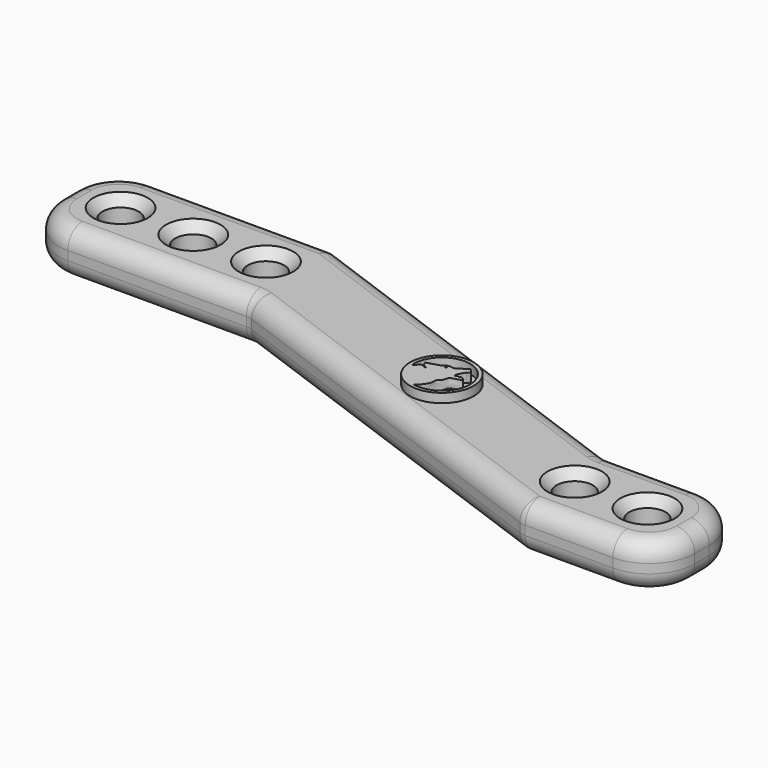
from build123d import *

# Parameters (mm, degrees)
F0_W         = 25
F0_H         = 12
F0_W_2       = 15
F1_DEPTH     = 5
F2_R         = 2
F3_DEPTH     = 5.001
F4_R         = 2
F5_T1_DEPTH  = 5
F5_T4_ANGLE  = 90
F5_T6_ANGLE  = 90
F5_T8_ANGLE  = 90
F5_T10_ANGLE = 90
F5_T12_ANGLE = 90
F5_T14_ANGLE = 90
F5_T16_ANGLE = 90
F5_T18_ANGLE = 90
F6_SIZE      = 1
F8_DEPTH     = 1


# Not quite as in the source:
# - a fillet or chamfer that OpenCascade refuses, or shapes differently, is made with other operations: its cross-section is extruded or revolved along the edge and cut away or added


with BuildPart() as f1:
    # F0 (on Top) → F1 (new body)
    with BuildSketch(Plane.XY):
        with Locations((12.5, 6)):
            Rectangle(F0_W, F0_H)
        with Locations((74.7861679354, -9.3909064497)):
            Rectangle(F0_W_2, F0_H)
        Polygon((25, 12), (25, 0), (67.2861679354, -15.3909064497), (67.2861679354, -3.3909064497), align=None)
    extrude(amount=F1_DEPTH)

    # F2 (on face) → F3 (cut, through all)
    with BuildSketch(Plane.XY.offset(5)):
        with Locations((6, 6)):
            Circle(F2_R)
        with Locations((14, 6)):
            Circle(F2_R)
        with Locations((22, 6)):
            Circle(F2_R)
        with Locations((68.2861679354, -9.3909064497)):
            Circle(F2_R)
        with Locations((76.2861679354, -9.3909064497)):
            Circle(F2_R)
    extrude(amount=-F3_DEPTH, mode=Mode.SUBTRACT)

    # F4
    f4_edges = [f1.edges().sort_by_distance(p)[0] for p in [
        (12.5, 12, 5),
        (12.5, 12, 0),
        (0, 6, 5),
        (0, 6, 0),
        (12.5, 0, 5),
        (12.5, 0, 0),
        (46.143084, -7.695453, 5),
        (74.786168, -15.390906, 5),
        (46.143084, -7.695453, 0),
        (74.786168, -15.390906, 0),
        (82.286168, -9.390906, 5),
        (82.286168, -9.390906, 0),
        (74.786168, -3.390906, 0),
        (74.786168, -3.390906, 5),
        (46.143084, 4.304547, 5),
        (46.143084, 4.304547, 0),
        (25, 12, 2.5),
        (67.286168, -3.390906, 2.5),
        (67.286168, -15.390906, 2.5),
        (25, 0, 2.5),
    ]]
    fillet(f4_edges, radius=F4_R)

    # F5: fillet of radius 5 on 6 edges, made by hand

    # F5_s2 → F5_t1 (cut)
    with BuildSketch(Plane.XY):
        with BuildLine():
            ThreePointArc((0, 5), (1.4644660941, 1.4644660941), (5, 0))
            Line((5, 0), (0, 0))
            Line((0, 0), (0, 5))
        make_face()
        with BuildLine():
            ThreePointArc((82.2861679354, -10.3909064497), (80.8217018413, -13.9264403556), (77.2861679354, -15.3909064497))
            Line((77.2861679354, -15.3909064497), (82.2861679354, -15.3909064497))
            Line((82.2861679354, -15.3909064497), (82.2861679354, -10.3909064497))
        make_face()
        with BuildLine():
            ThreePointArc((77.2861679354, -3.3909064497), (80.8217018413, -4.8553725437), (82.2861679354, -8.3909064497))
            Line((82.2861679354, -8.3909064497), (82.2861679354, -3.3909064497))
            Line((82.2861679354, -3.3909064497), (77.2861679354, -3.3909064497))
        make_face()
        with BuildLine():
            ThreePointArc((0, 7), (1.4644660941, 10.5355339059), (5, 12))
            Line((5, 12), (0, 12))
            Line((0, 12), (0, 7))
        make_face()
    extrude(amount=F5_T1_DEPTH, mode=Mode.SUBTRACT)

    # F5_s3 → F5_t4 (revolve, cut)
    with BuildSketch(Plane.XZ.offset(-5)):
        with BuildLine():
            ThreePointArc((2, 5), (0.5857864376, 4.4142135624), (0, 3))
            Line((0, 3), (0, 5))
            Line((0, 5), (2, 5))
        make_face()
    revolve(axis=Axis((5, 5, 5), (0, 0, 1)), revolution_arc=F5_T4_ANGLE, mode=Mode.SUBTRACT)

    # F5_s5 → F5_t6 (revolve, cut)
    with BuildSketch(Plane.YZ.offset(5)):
        with BuildLine():
            ThreePointArc((2, 0), (0.5857864376, 0.5857864376), (0, 2))
            Line((0, 2), (0, 0))
            Line((0, 0), (2, 0))
        make_face()
    revolve(axis=Axis((5, 5, 0), (0, 0, -1)), revolution_arc=F5_T6_ANGLE, mode=Mode.SUBTRACT)

    # F5_s7 → F5_t8 (revolve, cut)
    with BuildSketch(Plane.YZ.offset(5)):
        with BuildLine():
            ThreePointArc((10, 5), (11.4142135624, 4.4142135624), (12, 3))
            Line((12, 3), (12, 5))
            Line((12, 5), (10, 5))
        make_face()
    revolve(axis=Axis((5, 7, 5), (0, 0, 1)), revolution_arc=F5_T8_ANGLE, mode=Mode.SUBTRACT)

    # F5_s9 → F5_t10 (revolve, cut)
    with BuildSketch(Plane.XZ.offset(8.3909064497)):
        with BuildLine():
            ThreePointArc((80.2861679354, 5), (81.7003814977, 4.4142135624), (82.2861679354, 3))
            Line((82.2861679354, 3), (82.2861679354, 5))
            Line((82.2861679354, 5), (80.2861679354, 5))
        make_face()
    revolve(axis=Axis((77.2861679354, -8.3909064497, 5), (0, 0, 1)), revolution_arc=F5_T10_ANGLE, mode=Mode.SUBTRACT)

    # F5_s11 → F5_t12 (revolve, cut)
    with BuildSketch(Plane.YZ.offset(77.2861679354)):
        with BuildLine():
            ThreePointArc((-13.3909064497, 5), (-14.805120012, 4.4142135624), (-15.3909064497, 3))
            Line((-15.3909064497, 3), (-15.3909064497, 5))
            Line((-15.3909064497, 5), (-13.3909064497, 5))
        make_face()
    revolve(axis=Axis((77.2861679354, -10.3909064497, 5), (0, 0, 1)), revolution_arc=F5_T12_ANGLE, mode=Mode.SUBTRACT)

    # F5_s13 → F5_t14 (revolve, cut)
    with BuildSketch(Plane.XZ.offset(10.3909064497)):
        with BuildLine():
            ThreePointArc((80.2861679354, 0), (81.7003814977, 0.5857864376), (82.2861679354, 2))
            Line((82.2861679354, 2), (82.2861679354, 0))
            Line((82.2861679354, 0), (80.2861679354, 0))
        make_face()
    revolve(axis=Axis((77.2861679354, -10.3909064497, 0), (0, 0, -1)), revolution_arc=F5_T14_ANGLE, mode=Mode.SUBTRACT)

    # F5_s15 → F5_t16 (revolve, cut)
    with BuildSketch(Plane.YZ.offset(77.2861679354)):
        with BuildLine():
            ThreePointArc((-5.3909064497, 0), (-3.9766928873, 0.5857864376), (-3.3909064497, 2))
            Line((-3.3909064497, 2), (-3.3909064497, 0))
            Line((-3.3909064497, 0), (-5.3909064497, 0))
        make_face()
    revolve(axis=Axis((77.2861679354, -8.3909064497, 0), (0, 0, -1)), revolution_arc=F5_T16_ANGLE, mode=Mode.SUBTRACT)

    # F5_s17 → F5_t18 (revolve, cut)
    with BuildSketch(Plane.XZ.offset(-7)):
        with BuildLine():
            ThreePointArc((2, 0), (0.5857864376, 0.5857864376), (0, 2))
            Line((0, 2), (0, 0))
            Line((0, 0), (2, 0))
        make_face()
    revolve(axis=Axis((5, 7, 0), (0, 0, -1)), revolution_arc=F5_T18_ANGLE, mode=Mode.SUBTRACT)

    # F6
    f6_edges = [f1.edges().sort_by_distance(p)[0] for p in [
        (79.407488, -6.269586, 5),
        (80.286168, -9.390906, 5),
        (79.407488, -12.512227, 5),
        (72.462495, -13.390906, 5),
        (46.827124, -5.816068, 5),
        (25.341939, 1.939231, 5),
        (14.823673, 2, 5),
        (2.87868, 2.87868, 5),
        (2, 6, 5),
        (2.87868, 9.12132, 5),
        (14.823673, 10, 5),
        (45.459044, 2.425162, 5),
        (66.944229, -5.330137, 5),
        (72.462495, -5.390906, 5),
        (66.286168, -9.390906, 5),
        (74.286168, -9.390906, 5),
        (4, 6, 5),
        (12, 6, 5),
        (20, 6, 5),
    ]]
    chamfer(f6_edges, length=F6_SIZE)

    # F7 (on face) → F8 (join)
    with BuildSketch(Plane.XY.offset(5)):
        with BuildLine():
            ThreePointArc((51.5714465489, -2.3973205765), (46.0639290216, 0.4697115785), (46.8743760472, -5.6862447492))
            ThreePointArc((46.8743760472, -5.6862447492), (50.0789640761, -5.2643527315), (51.5714465489, -2.3973205765))
        make_face()
        with BuildLine():
            ThreePointArc((47.4314412964, -5.4305355832), (47.2191921032, -5.377867902), (47.0111841046, -5.3103677009))
            ThreePointArc((47.0111841046, -5.3103677009), (45.6038451401, -4.2737382506), (44.9810040585, -2.6405595815))
            ThreePointArc((44.9810040585, -2.6405595815), (47.9497331976, 0.7002891246), (51.1714465489, -2.3973205765))
            ThreePointArc((51.1714465489, -2.3973205765), (50.0241349159, -4.8050182613), (47.4314412964, -5.4305355832))
        make_face(mode=Mode.SUBTRACT)
        with BuildLine():
            ThreePointArc((44.9810040585, -2.6405595815), (45.6038451401, -4.2737382506), (47.0111841046, -5.3103677009))
            ThreePointArc((47.0111841046, -5.3103677009), (47.2191921032, -5.377867902), (47.4314412964, -5.4305355832))
            add(Edge.make_bspline(
                [(47.4314412964, -5.4305355832), (47.6314367313, -5.2519198305), (48.0362906471, -4.8872836094), (48.468150212, -4.0717796771), (48.2924237267, -3.5762982707), (48.9011177808, -3.2811798776), (48.8494271325, -2.4640809426), (49.8236616127, -2.3692057118), (50.2237885599, -2.0739698413), (49.9456305001, -1.8324852755), (49.5987799493, -1.8246132857), (49.4843735029, -1.9483257192), (49.3677026913, -1.8024479313), (49.3225296886, -1.9006184423), (48.8103474072, -2.0473285161), (49.581588425, -0.733870789), (49.5937064562, -0.9146074645), (49.6831355962, -0.8335828451), (49.6502679031, -0.7294239361), (49.7997941938, -0.6219848275), (49.6740369369, -0.4109902764), (49.5259184159, -0.1543038146), (49.3590367293, -0.1384905431), (48.0905454387, -1.0436348081), (48.026703291, -0.8670334883), (47.6419840925, -0.8347640081), (47.4018831656, -0.9005504349), (47.0836008469, -1.080456227), (47.1630236319, -1.2129956159), (45.5282289402, -1.5874370165), (45.6222497961, -1.6635138084), (45.6918513072, -1.7913162808), (45.739651642, -2.0224683846), (45.9078245747, -2.0914190074), (46.417628081, -2.3364929106), (45.9029191747, -2.2884877025), (45.8458841897, -2.1407284184), (45.5846462866, -2.0877978243), (45.3534270615, -2.3599985886), (45.1172854743, -2.5536514723), (45.0204691016, -2.6150925379), (44.9810040585, -2.6405595815)],
                knots=[0, 0, 0, 0, 0.042347164, 0.0857808372, 0.1160045286, 0.1501994234, 0.1877143295, 0.231240727, 0.2597008473, 0.2834528562, 0.310532914, 0.3272388783, 0.3435038371, 0.3571011567, 0.3789437154, 0.4283073163, 0.4370338972, 0.4498983608, 0.4646749244, 0.4819587762, 0.503796769, 0.5282983487, 0.5463726429, 0.6025425082, 0.6177409772, 0.6448745615, 0.6701858059, 0.6959492542, 0.7097201481, 0.7672938014, 0.7755739502, 0.7934281186, 0.8150112571, 0.836476617, 0.8637791999, 0.8885099845, 0.9073388771, 0.9284677792, 0.9558168743, 0.9817765779, 1, 1, 1, 1], degree=3))
        make_face()
        with BuildLine():
            add(Edge.make_bspline(
                [(47.3205000162, -1.299184165), (47.3170283076, -1.2970522608), (47.3309562262, -1.2738451866), (47.4421272866, -1.1822398815), (47.5953384947, -1.1176653509), (47.7620775243, -1.1526621903), (47.6142904797, -1.1898473793), (47.5352787361, -1.2182161742), (47.4398727725, -1.2649320685), (47.3293111063, -1.3045948726), (47.3205000162, -1.299184165)],
                knots=[0, 0, 0, 0, 0.0515685181, 0.1994645691, 0.3702317371, 0.4927206541, 0.6121771362, 0.7338439394, 0.86912068, 1, 1, 1, 1], degree=3))
        make_face(mode=Mode.SUBTRACT)
    extrude(amount=F8_DEPTH)


solid = f1.part
